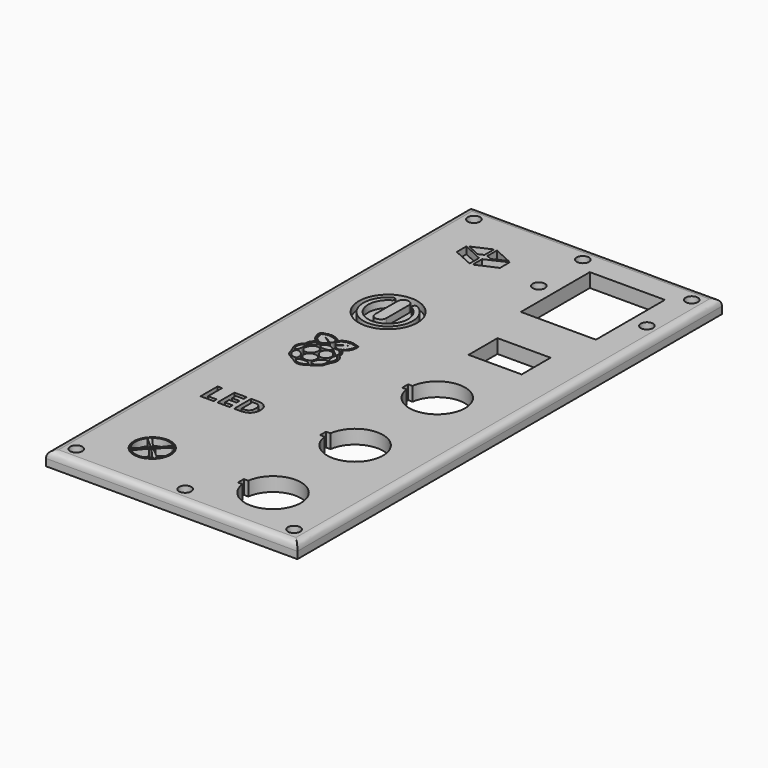
from build123d import *

# Parameters (mm, degrees)
F0_W         = 90
F0_H         = 190
F0_W_2       = 19
F0_H_2       = 12.9447032342
F0_W_3       = 26.885152871
F0_H_3       = 30.8681384815
F1_DEPTH     = 5
F3_D         = 4.4
F2_R         = 10.5
F2_R_2       = 6.6026154467
F2_R_3       = 6.3355773243
F2_R_4       = 6.05
F2_TEXT_SIZE = 10.6835823387
F2_R_5       = 0.67548
F4_DEPTH     = 2.5
F5_T1_DEPTH  = 202.5
F5_T3_DEPTH  = 102.5


# Not quite as in the source:
# - a fillet or chamfer that OpenCascade refuses, or shapes differently, is made with other operations: its cross-section is extruded or revolved along the edge and cut away or added
# - ends of sketch curves that miss each other by under 0.0002 mm in the source are joined
# - Text() gives the source's letters only with a copy of the font that has no kerning and outlines rounded to 1/6400 em; it was checked with that copy


with BuildPart() as f1:
    # F0 (on Top) → F1 (new body)
    with BuildSketch(Plane.XY):
        with Locations((22.75, 0)):
            Rectangle(F0_W, F0_H)
        with BuildLine():
            ThreePointArc((33.3339795578, -73.9671999834), (53.2458096108, -75.2921999834), (33.3339795578, -76.6171999834))
            Line((33.3339795578, -76.6171999834), (31.7458096108, -76.6171999834))
            Line((31.7458096108, -76.6171999834), (31.7458096108, -73.9671999834))
            Line((31.7458096108, -73.9671999834), (33.3339795578, -73.9671999834))
        make_face(mode=Mode.SUBTRACT)
        with BuildLine():
            ThreePointArc((33.338314127, -37.2171999834), (53.25014418, -38.5421999834), (33.338314127, -39.8671999834))
            Line((33.338314127, -39.8671999834), (31.75014418, -39.8671999834))
            Line((31.75014418, -39.8671999834), (31.75014418, -37.2171999834))
            Line((31.75014418, -37.2171999834), (33.338314127, -37.2171999834))
        make_face(mode=Mode.SUBTRACT)
        with BuildLine():
            ThreePointArc((33.338314127, -0.4627003242), (53.25014418, -1.7877003242), (33.338314127, -3.1127003242))
            Line((33.338314127, -3.1127003242), (31.75014418, -3.1127003242))
            Line((31.75014418, -3.1127003242), (31.75014418, -0.4627003242))
            Line((31.75014418, -0.4627003242), (33.338314127, -0.4627003242))
        make_face(mode=Mode.SUBTRACT)
        with Locations((43.3118191411, 30.4987983491)):
            Rectangle(F0_W_2, F0_H_2, mode=Mode.SUBTRACT)
        with Locations((42.4446412745, 68.869809007)):
            Rectangle(F0_W_3, F0_H_3, mode=Mode.SUBTRACT)
    extrude(amount=F1_DEPTH)

    # F3 (through all)
    with Locations(Plane.XY.offset(5)):
        with Locations((23.1020652264, 68.869809007), (61.7872180974, 68.869809007), (-16.25, 89), (22.75, 89), (61.75, 89), (61.75, -89), (22.75, -89), (-16.25, -89)):
            Hole(F3_D / 2)

    # F2 (on face) → F4 (cut)
    with BuildSketch(Plane.XY.offset(5)):
        with Locations((0, 30.2693031153)):
            Circle(F2_R)
        with BuildLine():
            ThreePointArc((4.4174279258, 37.9123217379), (0, 21.4415399137), (-4.4174279258, 37.9123217379))
            ThreePointArc((-4.4174279258, 37.9123217379), (-3.2534308308, 37.6010083727), (-3.564744196, 36.4370112777))
            ThreePointArc((-3.564744196, 36.4370112777), (0, 23.1455382989), (3.564744196, 36.4370112777))
            ThreePointArc((3.564744196, 36.4370112777), (3.2534308308, 37.6010083727), (4.4174279258, 37.9123217379))
        make_face(mode=Mode.SUBTRACT)
        with BuildLine():
            Line((-2.000000095, 27.0264472237), (-2.000000095, 37.0264472237))
            ThreePointArc((-2.000000095, 37.0264472237), (-9.5e-08, 39.0264472237), (1.999999905, 37.0264472237))
            Line((1.999999905, 37.0264472237), (1.999999905, 27.0264472237))
            ThreePointArc((1.999999905, 27.0264472237), (-9.5e-08, 25.0264472237), (-2.000000095, 27.0264472237))
        make_face(mode=Mode.SUBTRACT)
        Polygon((0.4129905471, -9.9638585935), (0.7692205471, -9.9012685935), (1.4261205471, -9.6472685935), (1.8280005471, -9.4037585935), (2.2184305471, -9.0959585935), (2.4147505471, -8.9466685935), (2.7132705471, -8.7953185935), (3.2494905471, -8.5364385935), (3.9699205471, -8.0854285935), (4.2494705471, -7.9007285935), (4.4165205471, -7.8002785935), (4.5436605471, -7.7324985935), (4.9540105471, -7.4972285935), (5.2028005471, -7.3036985935), (5.4607605471, -7.0623785935), (5.7434605471, -6.7426085935), (5.9765805471, -6.4007185935), (6.2028705471, -5.9312085935), (6.3518805471, -5.4202785935), (6.4196305471, -5.1545185935), (6.5436205471, -4.7568785935), (6.6442205471, -4.4511885935), (6.7013805471, -4.2638085935), (6.7423105471, -4.1170985935), (6.8154905471, -3.8973285935), (6.8807305471, -3.7768885935), (6.9737205471, -3.6445585935), (7.1108705471, -3.4414685935), (7.2425005471, -3.2055785935), (7.3881805471, -2.8863585935), (7.4925505471, -2.5804185935), (7.5433805471, -2.2993785935), (7.5656505471, -1.9650985935), (7.5526605471, -1.5288485935), (7.4933305471, -1.1607485935), (7.3615005471, -0.7562485935), (7.1284605471, -0.2762085935), (6.9991405471, -0.0799085935), (6.8332405471, 0.1299214065), (6.6039605471, 0.3770814065), (6.3965705471, 0.5540714065), (6.2021505471, 0.7606214065), (6.1430705471, 0.9558414065), (6.1145205471, 1.2493314065), (6.0134805471, 1.9326714065), (5.7870605471, 2.5414114065), (5.4973705471, 2.9981314065), (5.1187705471, 3.3988514065), (4.6518605471, 3.7425214065), (4.4937805471, 3.8399314065), (4.6870605471, 3.9276714065), (4.8913505471, 4.0561314065), (5.0326105471, 4.2681014065), (5.0806205471, 4.3244314065), (5.2234905471, 4.3936914065), (5.4708505471, 4.5411714065), (5.5896705471, 4.6748514065), (5.6627105471, 4.8240814065), (5.7063005471, 4.9209714065), (5.7869105471, 4.9997214065), (6.0102505471, 5.1957814065), (6.1254805471, 5.3662214065), (6.1928305471, 5.5365314065), (6.2317705471, 5.6617014065), (6.2575005471, 5.7114014065), (6.2912205471, 5.7468714065), (6.3609005471, 5.8081914065), (6.4259905471, 5.9066014065), (6.4890205471, 6.0582714065), (6.5138605471, 6.2065114065), (6.5315605471, 6.3412414065), (6.6262605471, 6.5215914065), (6.7422605471, 6.7486814065), (6.7619405471, 7.0112014065), (6.7629805471, 7.1060314065), (6.8230205471, 7.2583014065), (6.8986205471, 7.5021714065), (6.8403705471, 7.8015214065), (6.7999205471, 7.9039914065), (6.8079105471, 8.0052314065), (6.8388405471, 8.2409714065), (6.8195105471, 8.4022814065), (6.7727105471, 8.5293814065), (6.6035405471, 8.6795314065), (6.2835805471, 8.7620814065), (6.1663405471, 8.7742714065), (6.0726205471, 8.8311614065), (5.8741305471, 8.9690514065), (5.4915105471, 9.0478514065), (5.3057005471, 9.0675214065), (5.2325905471, 9.0842814065), (5.1772105471, 9.1104714065), (5.0139105471, 9.1960314065), (4.7437805471, 9.2482014065), (4.6306605471, 9.2641414065), (4.4853805471, 9.3145414065), (4.3694105471, 9.3537114065), (4.2224805471, 9.3758714065), (4.0276805471, 9.3775414065), (3.8690205471, 9.3471014065), (3.7920705471, 9.3320414065), (3.6900105471, 9.3633314065), (3.5859205471, 9.3960214065), (3.4511305471, 9.4096314065), (3.2683205471, 9.3996014065), (3.1131005471, 9.3592314065), (2.9817205471, 9.3237514065), (2.7388005471, 9.3121514065), (2.5252405471, 9.3055814065), (2.3375105471, 9.2352114065), (2.2107605471, 9.1781314065), (2.0704805471, 9.1717714065), (1.8208405471, 9.1542114065), (1.5166205471, 8.9714714065), (1.3820905471, 8.8624114065), (1.2319205471, 8.8277014065), (1.0177505471, 8.7607514065), (0.7043205471, 8.5102914065), (0.3492205471, 8.0642414065), (0.0627005471, 7.5217714065), (0.0062505471, 7.3938714065), (-0.0459394529, 7.3097614065), (-0.0566694529, 7.3024414065), (-0.0649994529, 7.3035014065), (-0.0715594529, 7.3156114065), (-0.0746194529, 7.3483314065), (-0.0822194529, 7.3861214065), (-0.1115894529, 7.4634314065), (-0.2389094529, 7.7218614065), (-0.3668694529, 7.9497914065), (-0.4978494529, 8.1616914065), (-0.6100194529, 8.3180414065), (-0.9492094529, 8.6540214065), (-1.1496294529, 8.7820814065), (-1.3162494529, 8.8277014065), (-1.4366694529, 8.8473814065), (-1.5088494529, 8.8913114065), (-1.6009494529, 8.9714714065), (-1.8362794529, 9.1291314065), (-2.1463594529, 9.1730214065), (-2.2536794529, 9.1747714065), (-2.4218894529, 9.2387014065), (-2.5769494529, 9.3009514065), (-2.6740594529, 9.3118114065), (-2.8058094529, 9.3066514065), (-2.9871094529, 9.3048714065), (-3.1597694529, 9.3514514065), (-3.4371294529, 9.4090914065), (-3.6267594529, 9.4034814065), (-3.7732494529, 9.3638914065), (-3.8572694529, 9.3341014065), (-3.9675794529, 9.3512614065), (-4.0937994529, 9.3743714065), (-4.2526594529, 9.3757414065), (-4.4322294529, 9.3545714065), (-4.5988694529, 9.2983414065), (-4.6834994529, 9.2592014065), (-4.7982394529, 9.2449314065), (-5.0061394529, 9.2245514065), (-5.2440494529, 9.1196914065), (-5.3353094529, 9.0732414065), (-5.5160494529, 9.0547114065), (-5.8025994529, 9.0243314065), (-6.0946394529, 8.8750714065), (-6.2239694529, 8.7929614065), (-6.3793994529, 8.7620814065), (-6.6281494529, 8.7084614065), (-6.7632594529, 8.6303514065), (-6.8570394529, 8.5293814065), (-6.9185794529, 8.3107814065), (-6.9203794529, 8.1451214065), (-6.8904694529, 8.0005614065), (-6.8768594529, 7.9184314065), (-6.9229194529, 7.7887814065), (-6.9838594529, 7.5680214065), (-6.9052994529, 7.2674314065), (-6.8492494529, 7.1318814065), (-6.8435994529, 6.9947514065), (-6.8313294529, 6.7947614065), (-6.6908594529, 6.5012814065), (-6.6259894529, 6.3819714065), (-6.5981894529, 6.2324814065), (-6.5596094529, 6.0171814065), (-6.3910994529, 5.7786314065), (-6.3092594529, 5.6835914065), (-6.2736294529, 5.5744914065), (-6.2432994529, 5.4393614065), (-6.1618694529, 5.2886814065), (-6.0069794529, 5.1049114065), (-5.8221294529, 4.9670314065), (-5.7788694529, 4.9325714065), (-5.7543394529, 4.8819214065), (-5.7166194529, 4.7506514065), (-5.6176994529, 4.6112514065), (-5.4369694529, 4.4556514065), (-5.2357394529, 4.3652114065), (-5.1614894529, 4.3279114065), (-5.0858294529, 4.2119814065), (-4.9353494529, 4.0283614065), (-4.7956094529, 3.9339914065), (-4.6486594529, 3.8777514065), (-4.6230194529, 3.8714714065), (-4.6026394529, 3.8623314065), (-4.5979294529, 3.8540914065), (-4.6013794529, 3.8430914065), (-4.6558294529, 3.7939214065), (-4.8399494529, 3.6675514065), (-5.0664194529, 3.4966914065), (-5.2981494529, 3.2884814065), (-5.5660594529, 3.0042814065), (-5.7617194529, 2.7407814065), (-6.0397194529, 2.1259714065), (-6.1467994529, 1.6849614065), (-6.2004494529, 1.2021514065), (-6.2195194529, 0.9798814065), (-6.2555994529, 0.8207814065), (-6.3428694529, 0.6721314065), (-6.4967494529, 0.5383014065), (-6.8107994529, 0.2579514065), (-7.0893894529, -0.0908785935), (-7.3786894529, -0.6115685935), (-7.5779694529, -1.1910985935), (-7.6292194529, -1.4799185935), (-7.6511894529, -1.7970185935), (-7.6368594529, -2.2028185935), (-7.5752794529, -2.5641985935), (-7.4037394529, -3.0418285935), (-7.0713194529, -3.6159985935), (-6.9204794529, -3.8511785935), (-6.8607494529, -3.9920085935), (-6.8087494529, -4.1691185935), (-6.7324994529, -4.4331385935), (-6.6146794529, -4.7887785935), (-6.5245294529, -5.0663485935), (-6.4710994529, -5.2556285935), (-6.4308294529, -5.4200985935), (-6.2202094529, -6.0697985935), (-5.8910994529, -6.6568085935), (-5.5304194529, -7.0909885935), (-5.1049594529, -7.4537485935), (-4.6241594529, -7.7330085935), (-4.4239294529, -7.8415485935), (-4.1399294529, -8.0259085935), (-3.5561094529, -8.4051785935), (-3.1728894529, -8.6168085935), (-2.8171194529, -8.7843685935), (-2.6516194529, -8.8573985935), (-2.5226594529, -8.9234985935), (-2.2623594529, -9.1189085935), (-1.9263094529, -9.3920785935), (-1.5545194529, -9.6214185935), (-1.0448594529, -9.8424685935), (-0.5127694529, -9.9751685935), (-0.4512094529, -9.9799785935), (-0.3454294529, -9.9830385935), (-0.1663294529, -9.9841985935), (0.0389705471, -9.9819885935), align=None)
        Polygon((-5.3410694529, -1.5345585935), (-5.3920194529, -1.9313085935), (-5.5290994529, -2.5204985935), (-5.6988994529, -3.0155285935), (-5.8435294529, -3.3077885935), (-5.9885094529, -3.4900685935), (-6.2103994529, -3.5682185935), (-6.3803994529, -3.5049785935), (-6.4895294529, -3.3949485935), (-6.6119494529, -3.2332685935), (-6.7888394529, -2.9339885935), (-6.9465694529, -2.5147385935), (-7.0255494529, -2.0679385935), (-7.0263494529, -1.6133885935), (-6.9276994529, -1.0946985935), (-6.7221794529, -0.6251985935), (-6.4666494529, -0.2841585935), (-6.1576894529, 0.0101914065), (-5.8992694529, 0.1806014065), (-5.7388994529, 0.2269814065), (-5.6127294529, 0.1952614065), (-5.5031794529, 0.1024814065), (-5.3728594529, -0.1579485935), (-5.3388494529, -0.3373085935), (-5.3190194529, -0.5917185935), (-5.3158194529, -1.0799485935), align=None, mode=Mode.SUBTRACT)
        Polygon((1.6861205471, -8.6820185935), (1.4279705471, -8.8863385935), (1.0098105471, -9.1302385935), (0.5948805471, -9.2889285935), (0.2614505471, -9.3569685935), (-0.0863594529, -9.3777285935), (-0.4294894529, -9.3593685935), (-0.6263694529, -9.3285285935), (-1.0649894529, -9.1739185935), (-1.4737994529, -8.9596685935), (-1.8212894529, -8.7097685935), (-2.0017294529, -8.5369485935), (-2.1326794529, -8.3659485935), (-2.2166894529, -8.1174885935), (-2.1828694529, -7.9693385935), (-2.0765794529, -7.8331885935), (-1.9374794529, -7.7296685935), (-1.7455994529, -7.6251785935), (-1.3067194529, -7.4544185935), (-0.8106094529, -7.3390885935), (0.0818905471, -7.2703785935), (0.8232505471, -7.3249685935), (1.4552405471, -7.4728985935), (1.7088205471, -7.5746585935), (1.9093705471, -7.6910885935), (2.0483305471, -7.8193085935), (2.1171405471, -7.9564385935), (2.1134005471, -8.0724285935), (2.0617505471, -8.2118085935), (1.8988105471, -8.4577985935), align=None, mode=Mode.SUBTRACT)
        Polygon((-2.5597894529, -6.4375885935), (-2.5740694529, -6.7531385935), (-2.6816894529, -7.0865085935), (-2.8851794529, -7.2913585935), (-3.1287594529, -7.3741085935), (-3.4593294529, -7.3977585935), (-3.7637494529, -7.3763885935), (-3.9623194529, -7.3371185935), (-4.4806294529, -7.1097085935), (-4.9705994529, -6.7541885935), (-5.2945294529, -6.4184885935), (-5.5313094529, -6.0603885935), (-5.7055194529, -5.6341285935), (-5.8251894529, -5.1737485935), (-5.8719594529, -4.8286685935), (-5.8698594529, -4.5312185935), (-5.7920494529, -4.1634985935), (-5.6496994529, -3.8915285935), (-5.4432894529, -3.7156885935), (-5.1184594529, -3.6323285935), (-4.7061294529, -3.6835585935), (-4.3614794529, -3.8184185935), (-3.9950394529, -4.0388485935), (-3.6343894529, -4.3222285935), (-3.2543494529, -4.7062785935), (-2.9659094529, -5.1093285935), (-2.7484194529, -5.5806585935), (-2.6077194529, -6.0728685935), align=None, mode=Mode.SUBTRACT)
        Polygon((2.2137405471, -4.9170285935), (2.1814605471, -5.1051185935), (2.0198905471, -5.5137185935), (1.7665305471, -5.8840385935), (1.4381205471, -6.2010385935), (0.9774205471, -6.4857485935), (0.4630505471, -6.6508885935), (0.2064805471, -6.6777185935), (-0.0947794529, -6.6805585935), (-0.3233694529, -6.6664685935), (-0.5127694529, -6.6384185935), (-1.0944194529, -6.4263185935), (-1.5859294529, -6.0748485935), (-1.8908794529, -5.7160685935), (-2.1096994529, -5.2968385935), (-2.1786794529, -5.0248485935), (-2.2128694529, -4.6936285935), (-2.2124094529, -4.4340285935), (-2.1854894529, -4.2092785935), (-2.0585994529, -3.8332485935), (-1.8460694529, -3.4825485935), (-1.5608294529, -3.1703885935), (-1.1488894529, -2.8699685935), (-0.6750494529, -2.6630985935), (-0.2585594529, -2.5828285935), (0.1904505471, -2.5793085935), (0.5421105471, -2.6294385935), (0.8733205471, -2.7253185935), (1.3630005471, -2.9945185935), (1.7772105471, -3.3860985935), (2.0233405471, -3.7509885935), (2.1782805471, -4.1429785935), (2.2177705471, -4.3952785935), (2.2273405471, -4.6915385935), align=None, mode=Mode.SUBTRACT)
        Polygon((-0.4757094529, -0.8893285935), (-0.5275094529, -1.1305885935), (-0.7128294529, -1.6005385935), (-0.9809594529, -2.0255685935), (-1.3190394529, -2.3925785935), (-1.7897594529, -2.7327985935), (-2.3186394529, -2.9527485935), (-2.5973394529, -3.0011885935), (-2.9215594529, -3.0162585935), (-3.1648094529, -3.0039685935), (-3.3626494529, -2.9698685935), (-3.8643194529, -2.7348185935), (-4.2709194529, -2.3510885935), (-4.5012694529, -1.9704785935), (-4.6349894529, -1.5406885935), (-4.6759394529, -1.1859985935), (-4.6645494529, -0.8491885935), (-4.5357494529, -0.2908785935), (-4.3541894529, 0.1158814065), (-4.0909794529, 0.5129414065), (-3.8461694529, 0.7916014065), (-3.5835594529, 1.0194014065), (-3.3775994529, 1.1511014065), (-3.1368694529, 1.2749114065), (-2.7684294529, 1.4146514065), (-2.4596294529, 1.4665114065), (-2.1201894529, 1.4719914065), (-1.8646394529, 1.4444914065), (-1.6453994529, 1.3895814065), (-1.1807094529, 1.1461114065), (-0.8156794529, 0.7879914065), (-0.6077794529, 0.4366514065), (-0.4766694529, 0.0322514065), (-0.4414694529, -0.2710585935), (-0.4458994529, -0.6186685935), align=None, mode=Mode.SUBTRACT)
        Polygon((4.5679205471, -0.6309085935), (4.5888605471, -0.8796585935), (4.5681105471, -1.3776085935), (4.4475105471, -1.8184685935), (4.2821805471, -2.1263385935), (4.0543005471, -2.4015685935), (3.6422605471, -2.7107985935), (3.1677205471, -2.8836985935), (2.7601505471, -2.9214285935), (2.3294305471, -2.8707985935), (1.8619505471, -2.7068285935), (1.4261105471, -2.4343785935), (1.0407005471, -2.0723285935), (0.6767605471, -1.5562785935), (0.4397405471, -0.9729085935), (0.3751205471, -0.6057485935), (0.3643805471, -0.2151185935), (0.3934005471, 0.0796814065), (0.4551105471, 0.3405814065), (0.6588005471, 0.7756114065), (0.9458905471, 1.1235014065), (1.3012405471, 1.3787314065), (1.7097005471, 1.5357814065), (2.1781005471, 1.5890214065), (2.6707905471, 1.5221414065), (3.1703505471, 1.3288014065), (3.5675905471, 1.0719114065), (3.9164505471, 0.7438014065), (4.1490305471, 0.4439114065), (4.3389105471, 0.1133914065), (4.4562505471, -0.1583085935), (4.5317305471, -0.4149485935), align=None, mode=Mode.SUBTRACT)
        Polygon((5.3340605471, -6.2315485935), (5.1853205471, -6.4262285935), (4.7090105471, -6.9116685935), (4.1696005471, -7.2536085935), (3.7215005471, -7.4108085935), (3.2683005471, -7.4611585935), (3.0619605471, -7.4486685935), (2.9351305471, -7.4296685935), (2.6626105471, -7.3244585935), (2.4783805471, -7.1506385935), (2.3882205471, -6.9569985935), (2.3401105471, -6.7058785935), (2.3406305471, -6.3746285935), (2.4004905471, -6.0032185935), (2.5135105471, -5.6115485935), (2.7065805471, -5.1509985935), (2.9548305471, -4.7225485935), (3.2757905471, -4.3314585935), (3.6910605471, -3.9337685935), (4.0296705471, -3.6653185935), (4.3353905471, -3.4751385935), (4.7294105471, -3.3402985935), (5.0782205471, -3.3454285935), (5.3051705471, -3.4455785935), (5.4781205471, -3.6286285935), (5.6199805471, -3.9338385935), (5.7109305471, -4.3054685935), (5.7490605471, -4.7155885935), (5.7235605471, -5.2103685935), (5.6188705471, -5.6740985935), (5.5376605471, -5.8894285935), (5.4406005471, -6.0743485935), align=None, mode=Mode.SUBTRACT)
        Polygon((6.7211005471, -2.2339085935), (6.5095705471, -2.8849085935), (6.3583605471, -3.1383885935), (6.1765305471, -3.3659085935), (6.0292805471, -3.5006585935), (5.9442905471, -3.5377385935), (5.8590905471, -3.5153585935), (5.7799905471, -3.4760385935), (5.6572105471, -3.3683485935), (5.5386205471, -3.1996985935), (5.3649405471, -2.8217185935), (5.2277705471, -2.3793285935), (5.1125105471, -1.8501685935), (5.0689205471, -1.5227485935), (5.0435405471, -1.1503885935), (5.0367505471, -0.7747685935), (5.0531505471, -0.3845985935), (5.0965405471, -0.1160585935), (5.1751005471, 0.0643514065), (5.2800905471, 0.2009214065), (5.3725005471, 0.2679714065), (5.4666605471, 0.2918914065), (5.6108205471, 0.2426114065), (5.7692805471, 0.1478714065), (6.0706505471, -0.0926885935), (6.4154305471, -0.5194585935), (6.6442805471, -1.0196185935), (6.7529805471, -1.5663285935), align=None, mode=Mode.SUBTRACT)
        Polygon((-2.3929794529, 3.4417714065), (-2.4590894529, 3.2531314065), (-2.5698594529, 3.0957614065), (-2.7678494529, 2.8675114065), (-3.1933694529, 2.4279214065), (-3.6203694529, 2.0234714065), (-4.0179694529, 1.6821514065), (-4.5492894529, 1.2798314065), (-4.9697794529, 1.0070814065), (-5.2231294529, 0.8833314065), (-5.4092694529, 0.8389614065), (-5.5058694529, 0.8580514065), (-5.5644494529, 0.9224314065), (-5.5810194529, 1.0271014065), (-5.5797094529, 1.1590714065), (-5.5512594529, 1.4579714065), (-5.5037494529, 1.7400614065), (-5.4419994529, 1.9794014065), (-5.3253094529, 2.2732414065), (-5.1801594529, 2.5302514065), (-4.8646694529, 2.9078114065), (-4.7045594529, 3.0598814065), (-4.5627794529, 3.1706214065), (-4.2938394529, 3.3214314065), (-3.9794194529, 3.4603814065), (-3.6979994529, 3.5409614065), (-3.4510694529, 3.5748314065), (-3.1416694529, 3.5921414065), (-2.8370494529, 3.5975814065), (-2.6188994529, 3.5873814065), (-2.5024294529, 3.5655214065), (-2.4296294529, 3.5291814065), align=None, mode=Mode.SUBTRACT)
        Polygon((1.7192405471, 3.2405114065), (1.8890505471, 3.0139314065), (1.9611805471, 2.8264014065), (1.9873605471, 2.6261714065), (1.9314105471, 2.3528214065), (1.6930605471, 2.0712214065), (1.3260805471, 1.8478814065), (0.8572905471, 1.6908014065), (0.2105305471, 1.6016114065), (-0.4965394529, 1.6286514065), (-0.7843394529, 1.6852814065), (-1.0937394529, 1.7796414065), (-1.3197494529, 1.8695114065), (-1.5045494529, 1.9645014065), (-1.8434594529, 2.2470414065), (-1.9433594529, 2.3702514065), (-2.0081994529, 2.4835614065), (-2.0502994529, 2.7857014065), (-1.9928794529, 3.0113414065), (-1.8924494529, 3.1531314065), (-1.7333794529, 3.3242114065), (-1.5923694529, 3.4535514065), (-1.4576594529, 3.5575914065), (-1.2271194529, 3.6902114065), (-0.9511994529, 3.8135514065), (-0.7308494529, 3.8921414065), (-0.5303194529, 3.9450114065), (-0.2112894529, 3.9832414065), (0.1303005471, 3.9797514065), (0.3902905471, 3.9488014065), (0.6231705471, 3.8939214065), (1.0732805471, 3.7085314065), (1.4709005471, 3.4604514065), align=None, mode=Mode.SUBTRACT)
        Polygon((-1.1066694529, 5.5427814065), (-1.4263794529, 5.7855714065), (-2.3201694529, 6.3897014065), (-3.0929894529, 6.8160314065), (-3.7615994529, 7.1237614065), (-4.0567694529, 7.2474514065), (-4.1488694529, 7.2819114065), (-4.1753294529, 7.2898214065), (-4.1829494529, 7.2911414065), (-4.1865594529, 7.2905814065), (-4.1867194529, 7.2901814065), (-4.1866094529, 7.2896314065), (-4.1855294529, 7.2880714065), (-4.1569694529, 7.2664114065), (-3.7643294529, 7.0316114065), (-3.0212394529, 6.5770814065), (-2.3194194529, 6.0904414065), (-1.8523794529, 5.7253814065), (-1.5046494529, 5.4079114065), (-1.3605894529, 5.2588714065), (-1.4164794529, 5.0815414065), (-1.5984994529, 4.7319314065), (-1.8994994529, 4.4357714065), (-2.2090994529, 4.2492614065), (-2.5746294529, 4.1104314065), (-2.9323994529, 4.0326514065), (-3.3302094529, 3.9814614065), (-3.6296894529, 3.9673214065), (-3.7826694529, 3.9817414065), (-3.8261294529, 4.0002014065), (-3.8354594529, 4.0190214065), (-3.8254394529, 4.0423714065), (-3.8044794529, 4.0655414065), (-3.7375894529, 4.1198514065), (-3.6731994529, 4.1792214065), (-3.6679994529, 4.1957514065), (-3.6743094529, 4.2098014065), (-3.7200194529, 4.2310414065), (-3.7896394529, 4.2445014065), (-3.9959194529, 4.2660914065), (-4.2415894529, 4.2965314065), (-4.4282794529, 4.3391214065), (-4.5466694529, 4.3893614065), (-4.5773294529, 4.4159514065), (-4.5874094529, 4.4427714065), (-4.5668194529, 4.4779014065), (-4.5047994529, 4.5111214065), (-4.4424694529, 4.5439214065), (-4.4275894529, 4.5579414065), (-4.4237094529, 4.5671114065), (-4.4278594529, 4.5733714065), (-4.4397294529, 4.5815514065), (-4.4833094529, 4.6022914065), (-4.6265594529, 4.6515814065), (-4.8367094529, 4.7239414065), (-5.0330994529, 4.8092514065), (-5.1783394529, 4.8894014065), (-5.2233994529, 4.9253014065), (-5.2350494529, 4.9463114065), (-5.2242994529, 4.9652114065), (-5.1948794529, 4.9850114065), (-5.0971194529, 5.0183614065), (-4.9591794529, 5.0480014065), (-5.2188294529, 5.1902514065), (-5.6021794529, 5.4343814065), (-5.7129394529, 5.5316914065), (-5.7400594529, 5.5679914065), (-5.7452594529, 5.5937114065), (-5.7363094529, 5.6047014065), (-5.7223794529, 5.6134014065), (-5.6852694529, 5.6281114065), (-5.5931694529, 5.6470614065), (-5.4532594529, 5.6632914065), (-5.6281394529, 5.7834714065), (-5.8097294529, 5.9215514065), (-5.9483494529, 6.0520314065), (-6.0400694529, 6.1719614065), (-6.0561194529, 6.2344814065), (-6.0477294529, 6.2486814065), (-6.0308094529, 6.2568814065), (-5.9698794529, 6.2532014065), (-5.8943694529, 6.2494714065), (-5.8392994529, 6.2606214065), (-5.8137894529, 6.2780214065), (-5.8154994529, 6.2979414065), (-5.8381094529, 6.3282714065), (-5.9568794529, 6.4364614065), (-6.1065194529, 6.5791514065), (-6.2246294529, 6.7198114065), (-6.2891394529, 6.8247614065), (-6.3060894529, 6.8847914065), (-6.2981894529, 6.9089714065), (-6.2694694529, 6.9222414065), (-6.1194694529, 6.9220614065), (-5.9328494529, 6.9097214065), (-6.1152794529, 7.0816614065), (-6.2588394529, 7.2298414065), (-6.3802294529, 7.3774014065), (-6.4496194529, 7.4823114065), (-6.4683694529, 7.5340114065), (-6.4647194529, 7.5396214065), (-6.4542794529, 7.5448514065), (-6.4159294529, 7.5537314065), (-6.2898594529, 7.5619414065), (-6.1551794529, 7.5718814065), (-6.1223594529, 7.5845314065), (-6.1116694529, 7.6025114065), (-6.1243594529, 7.6533814065), (-6.1488594529, 7.7168314065), (-6.2129394529, 7.8572814065), (-6.2787794529, 7.9837814065), (-6.3383794529, 8.0810014065), (-6.4031894529, 8.1886114065), (-6.4074194529, 8.2154914065), (-6.3985394529, 8.2362414065), (-6.3413794529, 8.2614214065), (-6.2543694529, 8.2713314065), (-5.9916894529, 8.2759614065), (-5.5799194529, 8.2759614065), (-5.6734094529, 8.3735414065), (-5.7319594529, 8.4489514065), (-5.7378894529, 8.4892014065), (-5.6806494529, 8.5302414065), (-5.5377094529, 8.5566314065), (-5.3600694529, 8.5538714065), (-5.1193894529, 8.5243014065), (-4.9356894529, 8.4894014065), (-4.7970694529, 8.4500414065), (-4.7573794529, 8.4479714065), (-4.7493694529, 8.4685414065), (-4.7590494529, 8.5033814065), (-4.8279694529, 8.5990714065), (-4.8824494529, 8.6785314065), (-4.8823894529, 8.7233114065), (-4.8195394529, 8.7401914065), (-4.6821394529, 8.7267914065), (-4.2466694529, 8.6194714065), (-4.1175194529, 8.5874114065), (-4.0828594529, 8.5835814065), (-4.0740694529, 8.5842914065), (-4.0703894529, 8.5859614065), (-4.0693794529, 8.5912614065), (-4.0725094529, 8.6004014065), (-4.0897594529, 8.6282214065), (-4.1581194529, 8.7080314065), (-4.2525794529, 8.8277014065), (-4.2607094529, 8.8562914065), (-4.2537694529, 8.8760814065), (-4.2078094529, 8.8896214065), (-4.1411994529, 8.8830714065), (-3.8883494529, 8.8125814065), (-3.6660094529, 8.7272214065), (-3.5418394529, 8.6666514065), (-3.4499894529, 8.6159714065), (-3.4220594529, 8.6038414065), (-3.4094294529, 8.6006414065), (-3.3964494529, 8.6045414065), (-3.3885994529, 8.6158414065), (-3.3872494529, 8.6541014065), (-3.3979594529, 8.6966314065), (-3.4412794529, 8.7905214065), (-3.4740794529, 8.8665414065), (-3.4787094529, 8.8950114065), (-3.4740594529, 8.9118314065), (-3.4510094529, 8.9183714065), (-3.4112294529, 8.9113314065), (-3.2923294529, 8.8619214065), (-2.9730594529, 8.6599814065), (-2.8185494529, 8.5592614065), (-2.7679794529, 8.5422914065), (-2.7338294529, 8.5478614065), (-2.7120794529, 8.5907214065), (-2.7214294529, 8.7116514065), (-2.7286994529, 8.8003914065), (-2.7202094529, 8.8210914065), (-2.7033694529, 8.8277014065), (-2.6818594529, 8.8222914065), (-2.6577594529, 8.8110214065), (-2.6020294529, 8.7778714065), (-2.4765394529, 8.6879114065), (-2.2521094529, 8.4907814065), (-2.1659594529, 8.4145714065), (-2.1335094529, 8.3952514065), (-2.1141794529, 8.3927314065), (-2.1065694529, 8.4025214065), (-2.1011494529, 8.4163914065), (-2.0931894529, 8.4519914065), (-2.0868694529, 8.5375214065), (-2.0756994529, 8.6357414065), (-2.0607694529, 8.6582914065), (-2.0387494529, 8.6654314065), (-2.0012994529, 8.6507414065), (-1.9568894529, 8.6193614065), (-1.8480194529, 8.5228614065), (-1.5743194529, 8.2353914065), (-1.4636494529, 8.1169214065), (-1.4340294529, 8.0886414065), (-1.4265494529, 8.0827014065), (-1.4244894529, 8.0815214065), (-1.4234394529, 8.0812314065), (-1.4203894529, 8.0832114065), (-1.4167094529, 8.0888814065), (-1.4080094529, 8.1097214065), (-1.3891494529, 8.1782214065), (-1.3596294529, 8.2608814065), (-1.3315194529, 8.2976714065), (-1.3183394529, 8.2992514065), (-1.2994194529, 8.2919814065), (-1.2467894529, 8.2536314065), (-1.0993694529, 8.1013414065), (-0.9279994529, 7.8855414065), (-0.7714394529, 7.6509714065), (-0.5414894529, 7.1721514065), (-0.4266694529, 6.7161914065), (-0.4207694529, 6.3934214065), (-0.4919394529, 6.1176714065), (-0.5951594529, 5.9465514065), (-0.7399594529, 5.7798114065), (-0.8645594529, 5.6712514065), (-0.9837794529, 5.5981914065), align=None, mode=Mode.SUBTRACT)
        Polygon((5.2979705471, 0.9843614065), (5.2830405471, 0.8663914065), (5.2312505471, 0.8001614065), (5.1419305471, 0.7788514065), (5.0130105471, 0.8025114065), (4.8424105471, 0.8711514065), (4.4496105471, 1.0996314065), (3.9845905471, 1.4341214065), (3.4914505471, 1.8348414065), (3.0143305471, 2.2620214065), (2.6427605471, 2.6282114065), (2.3478605471, 2.9569714065), (2.1895205471, 3.1713614065), (2.1116605471, 3.3327414065), (2.1037005471, 3.4070014065), (2.1107505471, 3.4539614065), (2.1323005471, 3.4771614065), (2.1650205471, 3.4932214065), (2.2836305471, 3.5224914065), (2.4510805471, 3.5415514065), (2.6519105471, 3.5501514065), (3.0917405471, 3.5350214065), (3.4792705471, 3.4751914065), (3.9251205471, 3.3166714065), (4.3179805471, 3.0879914065), (4.6524805471, 2.7942314065), (4.9644805471, 2.3713414065), (5.1791605471, 1.8733714065), (5.2447305471, 1.5768814065), (5.2876205471, 1.2365214065), align=None, mode=Mode.SUBTRACT)
        Polygon((5.0439005471, 4.8340914065), (4.6801205471, 4.6861414065), (4.4709005471, 4.6114414065), (4.4143405471, 4.5876014065), (4.3936705471, 4.5760314065), (4.3903305471, 4.5704214065), (4.3911405471, 4.5638114065), (4.4029205471, 4.5495314065), (4.4204605471, 4.5374914065), (4.4667005471, 4.5168414065), (4.5440305471, 4.4801514065), (4.5694905471, 4.4506414065), (4.5674405471, 4.4254214065), (4.5441305471, 4.4004314065), (4.4586705471, 4.3597814065), (4.3174905471, 4.3220014065), (3.9895605471, 4.2717514065), (3.7332305471, 4.2321414065), (3.6412805471, 4.1962514065), (3.6308605471, 4.1811714065), (3.6336105471, 4.1651214065), (3.6618105471, 4.1391614065), (3.7039005471, 4.1169014065), (3.7682105471, 4.0731314065), (3.7835705471, 4.0528314065), (3.7875905471, 4.0387714065), (3.7807605471, 4.0107514065), (3.7584805471, 3.9895114065), (3.6652705471, 3.9672614065), (3.5353805471, 3.9653114065), (3.3695505471, 3.9745914065), (3.1502705471, 3.9938114065), (2.5091805471, 4.1208714065), (1.9810705471, 4.3576714065), (1.6655405471, 4.6098014065), (1.4538805471, 4.9112414065), (1.3909905471, 5.0440214065), (1.3532905471, 5.1392814065), (1.3501505471, 5.2472714065), (1.4112505471, 5.3398414065), (1.5388505471, 5.4695414065), (2.0066305471, 5.8807114065), (2.6126805471, 6.3299914065), (3.1660805471, 6.6956314065), (3.7713605471, 7.0609314065), (4.1490305471, 7.2845114065), (4.1671205471, 7.2978714065), (4.1713205471, 7.3020914065), (4.1723005471, 7.3046714065), (4.1715705471, 7.3053514065), (4.1700405471, 7.3056314065), (4.1438005471, 7.2989014065), (3.7449405471, 7.1335714065), (3.0499005471, 6.8103014065), (2.3893205471, 6.4511114065), (1.4558305471, 5.8339814065), (1.2894305471, 5.7117414065), (1.1524705471, 5.6158714065), (1.0714305471, 5.5637214065), (1.0510105471, 5.5527514065), (1.0454105471, 5.5505514065), (1.0425505471, 5.5500014065), (0.9939405471, 5.5661914065), (0.9363705471, 5.5981814065), (0.8123305471, 5.6824114065), (0.7032805471, 5.7694114065), (0.6223305471, 5.8487214065), (0.4966405471, 6.0198814065), (0.4273405471, 6.1871414065), (0.4026005471, 6.3466114065), (0.3959805471, 6.5558214065), (0.4001605471, 6.7605814065), (0.4175005471, 6.9109914065), (0.4887805471, 7.1488314065), (0.6101505471, 7.4169714065), (0.7811905471, 7.7164114065), (0.9321105471, 7.9431514065), (1.0827005471, 8.1376114065), (1.2165005471, 8.2707914065), (1.2721005471, 8.3055114065), (1.3024305471, 8.3105914065), (1.3161805471, 8.3005914065), (1.3209705471, 8.2780714065), (1.3250705471, 8.2528114065), (1.3331405471, 8.2227514065), (1.3545905471, 8.1592914065), (1.3882205471, 8.0708514065), (1.6656305471, 8.3681414065), (1.7896405471, 8.4962114065), (1.8954405471, 8.5965914065), (1.9616305471, 8.6511414065), (1.9800005471, 8.6625814065), (1.9890105471, 8.6654314065), (2.0089405471, 8.6586714065), (2.0234305471, 8.6386114065), (2.0354905471, 8.5599514065), (2.0476705471, 8.4612714065), (2.0685605471, 8.4057814065), (2.0877105471, 8.3841714065), (2.1072505471, 8.3821814065), (2.1669805471, 8.4447714065), (2.2196605471, 8.5013414065), (2.3020605471, 8.5755814065), (2.4572205471, 8.7009514065), (2.5949805471, 8.7986814065), (2.6357805471, 8.8217014065), (2.6548605471, 8.8277014065), (2.6607405471, 8.8248314065), (2.6662105471, 8.8166114065), (2.6755105471, 8.7863914065), (2.6841005471, 8.6870614065), (2.6910905471, 8.5720014065), (2.6975105471, 8.5397814065), (2.7034105471, 8.5271214065), (2.7113605471, 8.5262414065), (2.7266705471, 8.5312314065), (2.7757205471, 8.5567114065), (2.9224805471, 8.6549514065), (3.1076705471, 8.7828014065), (3.2595605471, 8.8710014065), (3.4172005471, 8.9263314065), (3.4471505471, 8.9198314065), (3.4588705471, 8.8978314065), (3.4398305471, 8.8355114065), (3.3918605471, 8.7612614065), (3.3417305471, 8.6709514065), (3.3399105471, 8.6494014065), (3.3469805471, 8.6347214065), (3.3737005471, 8.6257614065), (3.4190505471, 8.6327714065), (3.5622805471, 8.6959614065), (3.7607505471, 8.7858014065), (3.9710005471, 8.8538614065), (4.1233105471, 8.8834614065), (4.1965905471, 8.8796114065), (4.2225205471, 8.8647614065), (4.2268405471, 8.8497914065), (4.2169405471, 8.8280814065), (4.1499605471, 8.7521014065), (4.0701005471, 8.6531214065), (4.0480205471, 8.5992514065), (4.0495205471, 8.5862714065), (4.0566505471, 8.5780714065), (4.0780005471, 8.5757114065), (4.1040305471, 8.5830314065), (4.2421405471, 8.6255514065), (4.4516805471, 8.6808514065), (4.6154105471, 8.7201914065), (4.7369105471, 8.7452914065), (4.8211405471, 8.7514314065), (4.8514405471, 8.7385914065), (4.8559305471, 8.7181514065), (4.8449905471, 8.6877514065), (4.7774805471, 8.5946014065), (4.7110805471, 8.5019614065), (4.7004505471, 8.4748314065), (4.7000705471, 8.4594614065), (4.7053705471, 8.4504914065), (4.7158805471, 8.4455014065), (4.7693705471, 8.4519414065), (5.0476305471, 8.5212514065), (5.2925505471, 8.5577514065), (5.6010405471, 8.5477814065), (5.6691005471, 8.5249314065), (5.6978105471, 8.4912214065), (5.6872605471, 8.4462414065), (5.6375605471, 8.3895514065), (5.5876805471, 8.3344914065), (5.5757605471, 8.3145914065), (5.5726505471, 8.3033914065), (5.5746605471, 8.3005914065), (5.5805605471, 8.2978814065), (5.6032305471, 8.2927414065), (5.9602005471, 8.2759614065), (6.1395905471, 8.2729514065), (6.2730505471, 8.2644314065), (6.3455605471, 8.2529414065), (6.3625205471, 8.2468314065), (6.3689705471, 8.2416314065), (6.3717105471, 8.2272814065), (6.3693605471, 8.2105514065), (6.3564005471, 8.1716214065), (6.3104005471, 8.0867414065), (6.1554505471, 7.8160414065), (6.0776905471, 7.6349614065), (6.0690505471, 7.5941514065), (6.0773505471, 7.5763214065), (6.1021005471, 7.5670614065), (6.1360605471, 7.5635114065), (6.2358005471, 7.5619414065), (6.3722305471, 7.5520114065), (6.4054405471, 7.5393614065), (6.4162805471, 7.5213714065), (6.3807305471, 7.4279714065), (6.3066105471, 7.3259514065), (6.0854905471, 7.0969714065), (5.8809705471, 6.9078814065), (6.0689705471, 6.9212514065), (6.2196405471, 6.9215014065), (6.2598305471, 6.9147414065), (6.2699305471, 6.9106114065), (6.2741005471, 6.9069114065), (6.2669305471, 6.8493414065), (6.2080905471, 6.7516314065), (5.9645005471, 6.4762514065), (5.8400005471, 6.3403214065), (5.8103405471, 6.2909514065), (5.8071005471, 6.2647914065), (5.8163605471, 6.2520414065), (5.8356905471, 6.2451314065), (5.9362405471, 6.2536714065), (6.0098505471, 6.2560914065), (6.0234205471, 6.2389814065), (6.0270205471, 6.2068014065), (6.0093905471, 6.1620614065), (5.9722805471, 6.1132914065), (5.8609905471, 6.0019314065), (5.5461505471, 5.7517014065), (5.4060705471, 5.6510014065), (5.5458805471, 5.6409214065), (5.6621005471, 5.6178614065), (5.6954405471, 5.5845314065), (5.6877205471, 5.5453214065), (5.6587405471, 5.5070314065), (5.5177505471, 5.3943614065), (5.2965305471, 5.2572014065), (5.1182705471, 5.1590214065), (4.9073105471, 5.0515714065), (5.0469805471, 5.0166414065), (5.1465805471, 4.9824514065), (5.1776105471, 4.9646214065), (5.1898805471, 4.9492714065), (5.1524805471, 4.9000914065), align=None, mode=Mode.SUBTRACT)
        with Locations((0, -75.2921999834)):
            Circle(F2_R_2)
        with Locations((0, -75.2921999834)):
            Circle(F2_R_3, mode=Mode.SUBTRACT)
        with Locations((0, -75.2921999834)):
            Circle(F2_R_4)
        with BuildLine():
            ThreePointArc((0.8504457784, -74.8269068219), (0.939198166, -75.0520696999), (0.96941, -75.2921999834))
            ThreePointArc((0.96941, -75.2921999834), (0.939198166, -75.5323302668), (0.8504457784, -75.7574931449))
            Line((0.8504457784, -75.7574931449), (4.24264, -78.5719699834))
            ThreePointArc((4.24264, -78.5719699834), (4.242643652, -79.5348436354), (3.2797713481, -79.5348386354))
            Line((3.2797713481, -79.5348386354), (0.46529, -76.1426399834))
            ThreePointArc((0.46529, -76.1426399834), (0, -76.2616099834), (-0.4652931615, -76.1426457618))
            Line((-0.4652931615, -76.1426457618), (-3.27977, -79.5348399834))
            ThreePointArc((-3.27977, -79.5348399834), (-4.242643652, -79.5348436354), (-4.242638652, -78.5719713315))
            Line((-4.242638652, -78.5719713315), (-0.85044, -75.7574899834))
            ThreePointArc((-0.85044, -75.7574899834), (-0.96941, -75.2921999834), (-0.8504457784, -74.8269068219))
            Line((-0.8504457784, -74.8269068219), (-4.24264, -72.0124299834))
            ThreePointArc((-4.24264, -72.0124299834), (-4.242643652, -71.0495563314), (-3.2797713481, -71.0495613314))
            Line((-3.2797713481, -71.0495613314), (-0.46529, -74.4417599834))
            ThreePointArc((-0.46529, -74.4417599834), (0, -74.3227899834), (0.4652931615, -74.441754205))
            Line((0.4652931615, -74.441754205), (3.27977, -71.0495599834))
            ThreePointArc((3.27977, -71.0495599834), (4.242643652, -71.0495563314), (4.242638652, -72.0124286353))
            Line((4.242638652, -72.0124286353), (0.8504457784, -74.8269068219))
        make_face(mode=Mode.SUBTRACT)
        Polygon((0.5772789161, 67.4277466968), (7.7962766649, 70.5836958078), (7.7962766649, 74.9680101871), (0.5772789161, 71.6230814777), align=None)
        Polygon((-0.4999009765, 71.6230814777), (-7.6999994926, 74.9680101871), (-7.6999994926, 70.6025950404), (-0.4999009765, 67.3899524742), align=None)
        Polygon((0.5157593575, 78.3618617952), (0.5157593575, 74.0430233184), (2.3832131351, 73.209776961), (7.0516651418, 75.372730392), align=None)
        Polygon((-0.4814684439, 74.0430233184), (-0.4814684439, 78.2944406017), (-7.020233827, 75.372730392), (-2.3186418705, 73.1913401857), align=None)
        with Locations((-10, -42.3882896253)):
            Text('LED', F2_TEXT_SIZE, font='Open Sans', font_style=FontStyle.BOLD, text_align=(TextAlign.LEFT, TextAlign.BOTTOM))
        with Locations((0, -75.2921999834)):
            Circle(F2_R_5)
    extrude(amount=-F4_DEPTH, mode=Mode.SUBTRACT)

    # F5: fillet of radius 2.5 on 4 edges, made by hand

    # F5_s2 → F5_t1 (cut)
    with BuildSketch(Plane.XZ.offset(-101.25)):
        with BuildLine():
            add(Edge.make_bspline(
                [(-22.25, 2.5), (-22.25, 5), (-19.75, 5)],
                knots=[0, 0, 0, 1, 1, 1], degree=2, weights=[1, 1, 1]))
            Line((-19.75, 5), (-22.25, 5))
            Line((-22.25, 5), (-22.25, 2.5))
        make_face()
        with BuildLine():
            add(Edge.make_bspline(
                [(65.25, 5), (67.75, 5), (67.75, 2.5)],
                knots=[0, 0, 0, 1, 1, 1], degree=2, weights=[1, 1, 1]))
            Line((67.75, 2.5), (67.75, 5))
            Line((67.75, 5), (65.25, 5))
        make_face()
    extrude(amount=F5_T1_DEPTH, mode=Mode.SUBTRACT)

    # F5_s4 → F5_t3 (cut)
    with BuildSketch(Plane.YZ.offset(-28.5)):
        with BuildLine():
            add(Edge.make_bspline(
                [(-95, 2.5), (-95, 5), (-92.5, 5)],
                knots=[0, 0, 0, 1, 1, 1], degree=2, weights=[1, 1, 1]))
            Line((-92.5, 5), (-95, 5))
            Line((-95, 5), (-95, 2.5))
        make_face()
        with BuildLine():
            add(Edge.make_bspline(
                [(95, 2.5), (95, 5), (92.5, 5)],
                knots=[0, 0, 0, 1, 1, 1], degree=2, weights=[1, 1, 1]))
            Line((92.5, 5), (95, 5))
            Line((95, 5), (95, 2.5))
        make_face()
    extrude(amount=F5_T3_DEPTH, mode=Mode.SUBTRACT)


solid = f1.part
